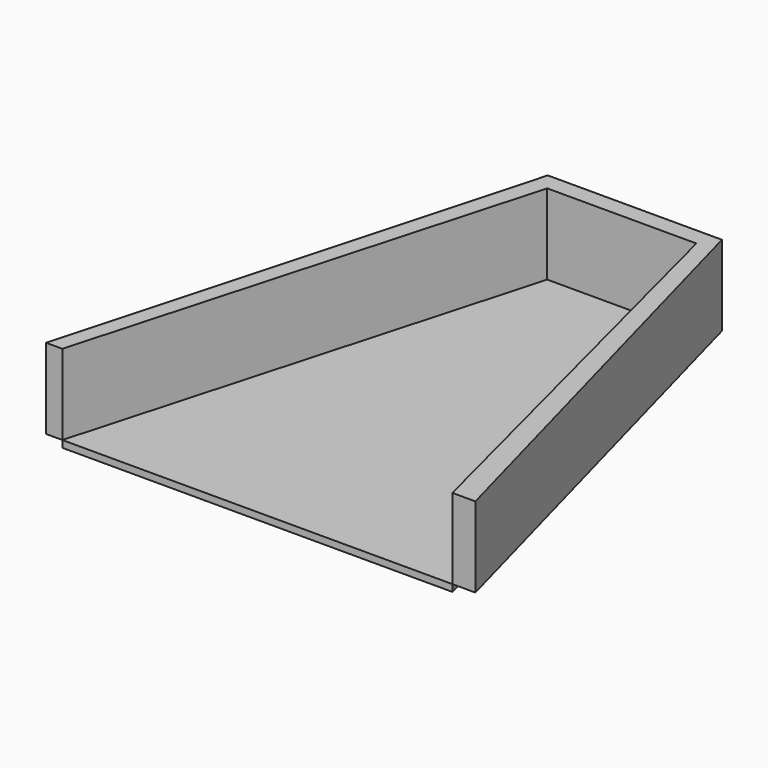
from build123d import *

# Parameters (mm, degrees)
F1_DEPTH = 3
F3_DEPTH = 343
F5_DEPTH = 35


# Not quite as in the source:
# - an extrude ends at something that could not be found from the text; its depth is read off the source's solid


with BuildPart() as f1:
    # F0 (on Top) → F1 (new body)
    with BuildSketch(Plane.XY):
        Polygon((30, 195.4140751933), (-35, 195.4140751933), (-90, 0), (0, 0), (80, 0), align=None)
    extrude(amount=F1_DEPTH)

    # F2 (on Top) → F3 (cut, through all)
    with BuildSketch(Plane.XY):
        with BuildLine():
            ThreePointArc((0, 109.7888334103), (7.3847296102, 112.8476885693), (10.4435847692, 120.2324181795))
            ThreePointArc((10.4435847692, 120.2324181795), (-7.3847296102, 127.6171477897), (0, 109.7888334103))
        make_face()
    extrude(amount=-F3_DEPTH, mode=Mode.SUBTRACT)


with BuildPart() as f5:
    # F4 (on face) → F5 (new body)
    with BuildSketch(Plane.XY.offset(3)):
        Polygon((-40.8189669251, 202.9922008514), (-97.0825403929, 0), (-90, 0), (-35, 195.4140751933), (30, 195.4140751933), (80, 0), (90.0265499949, 0), (35.0714325905, 202.9922008514), align=None)
    extrude(amount=F5_DEPTH)


solid = Compound([f1.part, f5.part])
